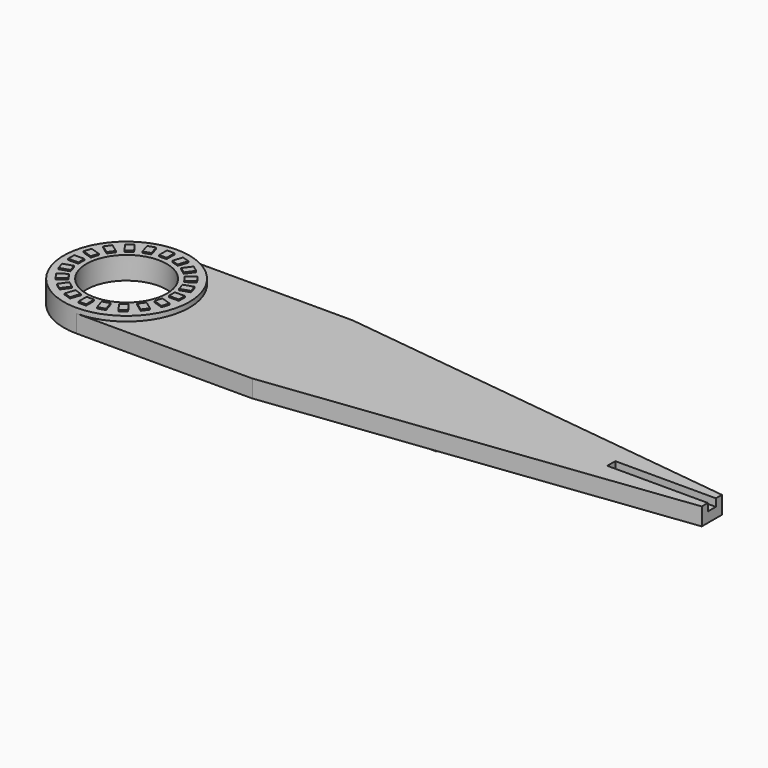
from build123d import *

# Parameters (mm, degrees)
F0_R         = 8
F1_DEPTH     = 3.5
F2_R         = 12.5
F2_R_2       = 8
F3_DEPTH     = 1
F4_W         = 1.5
F4_H         = 2
F4_W_2       = 2
F4_H_2       = 1.5
F5_DEPTH     = 0.25
F6_W         = 20
F6_H         = 2
F7_DEPTH     = 1.5
F8_TEXT_SIZE = 16.6975001186
F9_DEPTH     = 1.5


# Not quite as in the source:
# - Text() gives the source's letters only with a copy of the font that has no kerning and outlines rounded to 1/6400 em; it was checked with that copy


with BuildPart() as f1:
    # F0 (on Top) → F1 (new body)
    with BuildSketch(Plane.XY):
        with BuildLine():
            ThreePointArc((0, -12.5), (8.8388347648, -8.8388347648), (12.5, 0))
            ThreePointArc((12.5, 0), (8.8388347648, 8.8388347648), (0, 12.5))
            ThreePointArc((0, 12.5), (-12.5, 0), (0, -12.5))
        make_face()
        Circle(F0_R, mode=Mode.SUBTRACT)
        with BuildLine():
            ThreePointArc((0, 12.5), (8.8388347648, 8.8388347648), (12.5, 0))
            ThreePointArc((12.5, 0), (8.8388347648, -8.8388347648), (0, -12.5))
            Line((0, -12.5), (35, -12.5))
            Line((35, -12.5), (116.3887844346, -2.5067138408))
            Line((116.3887844346, -2.5067138408), (116.3887844346, 2.5067138408))
            Line((116.3887844346, 2.5067138408), (35, 12.5))
            Line((35, 12.5), (0, 12.5))
        make_face()
    extrude(amount=F1_DEPTH)

    # F2 (on face) → F3 (join)
    with BuildSketch(Plane.XY.offset(3.5)):
        Circle(F2_R)
        Circle(F2_R_2, mode=Mode.SUBTRACT)
    extrude(amount=F3_DEPTH)

    # F4 (on face) → F5 (join)
    with BuildSketch(Plane.XY.offset(4.5)):
        with Locations((0, 10)):
            Rectangle(F4_W, F4_H)
        Polygon((-2.6858945509, 10.693384425), (-4.1124793253, 10.2298589335), (-3.4944453366, 8.3277459009), (-2.0678605622, 8.7912713924), align=None)
        Polygon((-5.8588750294, 9.3400258773), (-7.072400521, 8.4583479989), (-5.8968300164, 6.8403140102), (-4.6833045249, 7.7219918886), align=None)
        Polygon((-8.4583479989, 7.072400521), (-9.3400258773, 5.8588750294), (-7.7219918886, 4.6833045249), (-6.8403140102, 5.8968300164), align=None)
        Polygon((-10.2298589335, 4.1124793253), (-10.693384425, 2.6858945509), (-8.7912713924, 2.0678605622), (-8.3277459009, 3.4944453366), align=None)
        with Locations((-10, 0)):
            Rectangle(F4_W_2, F4_H_2)
        Polygon((-10.693384425, -2.6858945509), (-10.2298589335, -4.1124793253), (-8.3277459009, -3.4944453366), (-8.7912713924, -2.0678605622), align=None)
        Polygon((-9.3400258773, -5.8588750294), (-8.4583479989, -7.072400521), (-6.8403140102, -5.8968300164), (-7.7219918886, -4.6833045249), align=None)
        Polygon((-7.072400521, -8.4583479989), (-5.8588750294, -9.3400258773), (-4.6833045249, -7.7219918886), (-5.8968300164, -6.8403140102), align=None)
        Polygon((-4.1124793253, -10.2298589335), (-2.6858945509, -10.693384425), (-2.0678605622, -8.7912713924), (-3.4944453366, -8.3277459009), align=None)
        with Locations((0, -10)):
            Rectangle(F4_W, F4_H)
        Polygon((2.6858945509, -10.693384425), (4.1124793253, -10.2298589335), (3.4944453366, -8.3277459009), (2.0678605622, -8.7912713924), align=None)
        Polygon((5.8588750294, -9.3400258773), (7.072400521, -8.4583479989), (5.8968300164, -6.8403140102), (4.6833045249, -7.7219918886), align=None)
        Polygon((8.4583479989, -7.072400521), (9.3400258773, -5.8588750294), (7.7219918886, -4.6833045249), (6.8403140102, -5.8968300164), align=None)
        Polygon((10.2298589335, -4.1124793253), (10.693384425, -2.6858945509), (8.7912713924, -2.0678605622), (8.3277459009, -3.4944453366), align=None)
        with Locations((10, 0)):
            Rectangle(F4_W_2, F4_H_2)
        Polygon((10.693384425, 2.6858945509), (10.2298589335, 4.1124793253), (8.3277459009, 3.4944453366), (8.7912713924, 2.0678605622), align=None)
        Polygon((9.3400258773, 5.8588750294), (8.4583479989, 7.072400521), (6.8403140102, 5.8968300164), (7.7219918886, 4.6833045249), align=None)
        Polygon((7.072400521, 8.4583479989), (5.8588750294, 9.3400258773), (4.6833045249, 7.7219918886), (5.8968300164, 6.8403140102), align=None)
        Polygon((4.1124793253, 10.2298589335), (2.6858945509, 10.693384425), (2.0678605622, 8.7912713924), (3.4944453366, 8.3277459009), align=None)
    extrude(amount=F5_DEPTH)

    # F6 (on face) → F7 (cut)
    with BuildSketch(Plane.XY.offset(3.5)):
        with Locations((106.3887844346, 0.0067138408)):
            Rectangle(F6_W, F6_H)
    extrude(amount=-F7_DEPTH, mode=Mode.SUBTRACT)

    # F8 (on face) → F9 (join)
    with BuildSketch(Plane(origin=(0, 0, 0), x_dir=(1, 0, 0), z_dir=(0, 0, -1))):
        with Locations((11.6528718383, -5.5987801453)):
            Text('RANDY', F8_TEXT_SIZE, font='Open Sans', text_align=(TextAlign.LEFT, TextAlign.BOTTOM))
    extrude(amount=F9_DEPTH)


solid = f1.part
